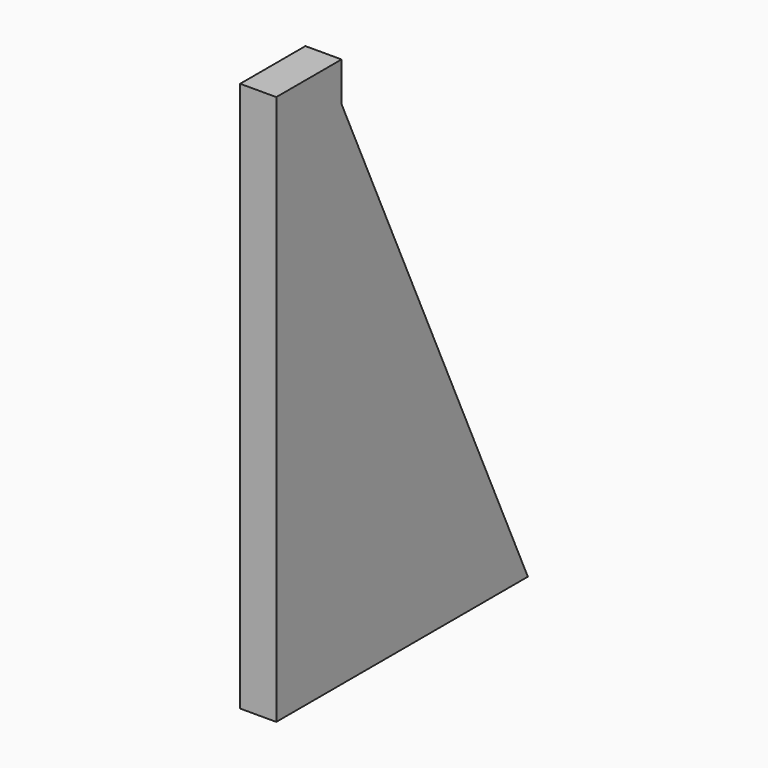
from build123d import *

# Parameters (mm, degrees)
F1_DEPTH = 4.7625


# Not quite as in the source:
# - a length typed as a fraction of an inch, garbled in the dataset ("3 / 203.2 mm" for 3/8 in), is restored


with BuildPart() as f1:
    # F0 (on Right) → F1 (new body, symmetric)
    with BuildSketch(Plane.YZ):
        Polygon((21.5, 62.8277051401), (0, 62.8277051401), (0, -82.1722948599), (82.89, -82.1722948599), (21.5, 52.4577051401), align=None)
    extrude(amount=F1_DEPTH, both=True)


solid = f1.part
